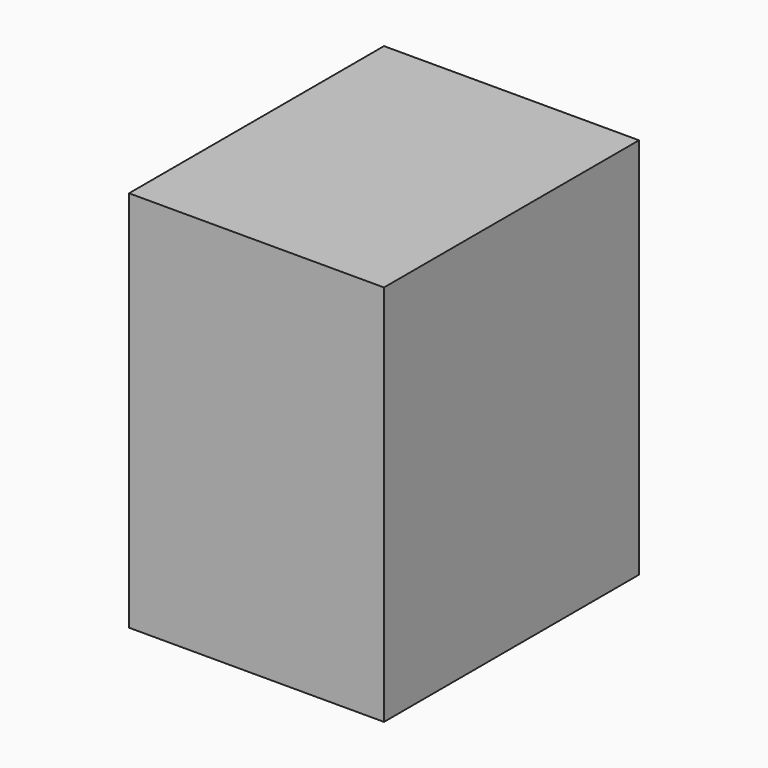
from build123d import *

# Parameters (mm, degrees)
F0_W     = 50.8
F0_H     = 76.2
F1_DEPTH = 31.75


# Not quite as in the source:
# - the program builds the solid bodies; features that only make, move or delete a surface that nothing else refers to are left out


with BuildPart() as f1:
    # F0 (on Front) → F1 (new body, symmetric)
    with BuildSketch(Plane.XZ):
        with Locations((25.4, 38.1)):
            Rectangle(F0_W, F0_H)
    extrude(amount=F1_DEPTH, both=True)


solid = f1.part
